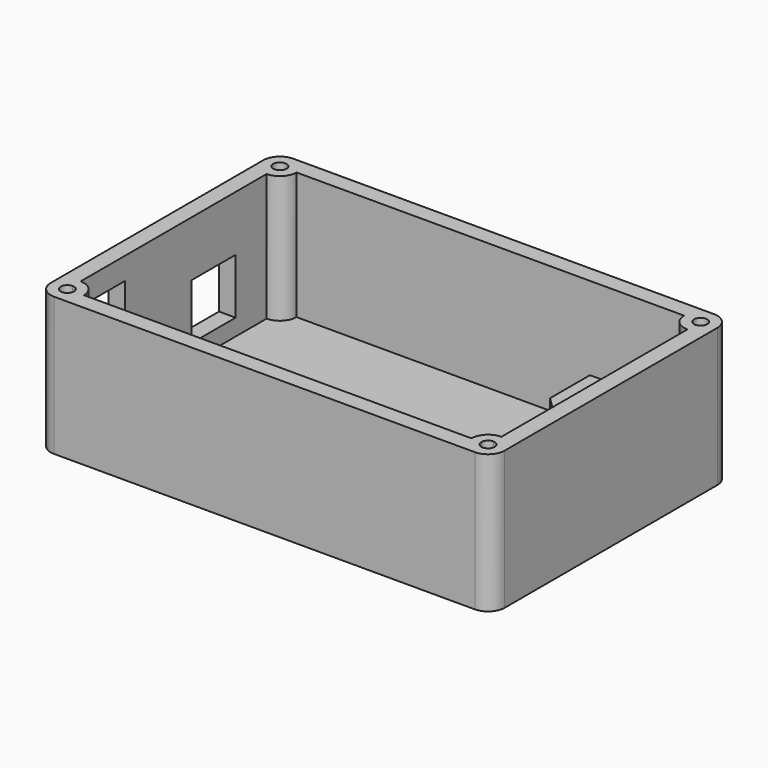
from build123d import *

# Parameters (mm, degrees)
F0_W     = 104.14
F0_H     = 68.58
F1_DEPTH = 31.75
F2_DEPTH = 12.7
F3_DEPTH = 2.54
F4_W     = 12.7
F4_H     = 12.7
F4_W_2   = 11.43
F4_H_2   = 20.32
F5_DEPTH = 10.16
F6_R     = 3.81
F7_R     = 3.80999
F8_DEPTH = 12.7


# Not quite as in the source:
# - a fillet or chamfer is up to 0.001 mm smaller than in the source, because OpenCascade refuses the exact size


with BuildPart() as f1:
    # F0 (on Top) → F1 (new body)
    with BuildSketch(Plane.XY):
        Rectangle(F0_W, F0_H)
        with BuildLine():
            ThreePointArc((-48.26, 28.956), (-49.3376307345, 31.5576307345), (-46.736, 30.48))
            Line((-46.736, 30.48), (-44.45, 30.48))
            Line((-44.45, 30.48), (22.86, 30.48))
            Line((22.86, 30.48), (25.4, 30.48))
            Line((25.4, 30.48), (44.45, 30.48))
            Line((44.45, 30.48), (46.736, 30.48))
            ThreePointArc((46.736, 30.48), (48.26, 32.004), (49.784, 30.48))
            ThreePointArc((49.784, 30.48), (49.3376307345, 29.4023692655), (48.26, 28.956))
            Line((48.26, 28.956), (48.26, 26.67))
            Line((48.26, 26.67), (48.26, -26.67))
            Line((48.26, -26.67), (48.26, -28.956))
            ThreePointArc((48.26, -28.956), (49.3376307345, -29.4023692655), (49.784, -30.48))
            ThreePointArc((49.784, -30.48), (48.26, -32.004), (46.736, -30.48))
            Line((46.736, -30.48), (44.45, -30.48))
            Line((44.45, -30.48), (25.4, -30.48))
            Line((25.4, -30.48), (22.86, -30.48))
            Line((22.86, -30.48), (-44.45, -30.48))
            Line((-44.45, -30.48), (-46.736, -30.48))
            ThreePointArc((-46.736, -30.48), (-49.3376307345, -31.5576307345), (-48.26, -28.956))
            Line((-48.26, -28.956), (-48.26, -26.67))
            Line((-48.26, -26.67), (-48.26, 26.67))
            Line((-48.26, 26.67), (-48.26, 28.956))
        make_face(mode=Mode.SUBTRACT)
        with BuildLine():
            Line((46.736, 30.48), (44.45, 30.48))
            Line((44.45, 30.48), (44.45, 26.67))
            Line((44.45, 26.67), (48.26, 26.67))
            Line((48.26, 26.67), (48.26, 28.956))
            ThreePointArc((48.26, 28.956), (47.1823692655, 29.4023692655), (46.736, 30.48))
        make_face()
        with BuildLine():
            Line((48.26, -28.956), (48.26, -26.67))
            Line((48.26, -26.67), (44.45, -26.67))
            Line((44.45, -26.67), (44.45, -30.48))
            Line((44.45, -30.48), (46.736, -30.48))
            ThreePointArc((46.736, -30.48), (47.1823692655, -29.4023692655), (48.26, -28.956))
        make_face()
        with BuildLine():
            Line((-44.45, -26.67), (-48.26, -26.67))
            Line((-48.26, -26.67), (-48.26, -28.956))
            ThreePointArc((-48.26, -28.956), (-47.1823692655, -29.4023692655), (-46.736, -30.48))
            Line((-46.736, -30.48), (-44.45, -30.48))
            Line((-44.45, -30.48), (-44.45, -26.67))
        make_face()
        with BuildLine():
            Line((-44.45, 30.48), (-46.736, 30.48))
            ThreePointArc((-46.736, 30.48), (-47.1823692655, 29.4023692655), (-48.26, 28.956))
            Line((-48.26, 28.956), (-48.26, 26.67))
            Line((-48.26, 26.67), (-44.45, 26.67))
            Line((-44.45, 26.67), (-44.45, 30.48))
        make_face()
    extrude(amount=F1_DEPTH)

    # F0 (on Top) → F2 (join)
    with BuildSketch(Plane.XY):
        Polygon((25.4, 30.48), (22.86, 30.48), (22.86, 19.05), (26.67, 15.24), (26.67, -24.13), (22.86, -27.94), (22.86, -30.48), (25.4, -30.48), (25.4, -27.94), (29.21, -24.13), (29.21, 15.24), (25.4, 19.05), align=None)
    extrude(amount=F2_DEPTH)

    # F0 (on Top) → F3 (join)
    with BuildSketch(Plane.XY):
        Polygon((22.86, 30.48), (-44.45, 30.48), (-44.45, 26.67), (-48.26, 26.67), (-48.26, -26.67), (-44.45, -26.67), (-44.45, -30.48), (22.86, -30.48), (22.86, -27.94), (26.67, -24.13), (26.67, 15.24), (22.86, 19.05), align=None)
        Polygon((44.45, 30.48), (25.4, 30.48), (25.4, 19.05), (29.21, 15.24), (29.21, -24.13), (25.4, -27.94), (25.4, -30.48), (44.45, -30.48), (44.45, -26.67), (48.26, -26.67), (48.26, 26.67), (44.45, 26.67), align=None)
    extrude(amount=F3_DEPTH)

    # F4 (on face) → F5 (cut)
    with BuildSketch(Plane(origin=(-52.07, 0, 0), x_dir=(0, -1, 0), z_dir=(-1, 0, 0))):
        with Locations((-11.43, 12.7)):
            Rectangle(F4_W, F4_H)
        with Locations((19.685, 16.51)):
            Rectangle(F4_W_2, F4_H_2)
    extrude(amount=-F5_DEPTH, mode=Mode.SUBTRACT)

    # F6
    f6_edges = [f1.edges().sort_by_distance(p)[0] for p in [
        (-52.07, -34.29, 15.875),
        (52.07, -34.29, 15.875),
        (52.07, 34.29, 15.875),
        (-52.07, 34.29, 15.875),
    ]]
    fillet(f6_edges, radius=F6_R)

    # F7 (radius 3.81 in the source; OpenCascade refuses exactly that, so slightly less here)
    f7_edges = [f1.edges().sort_by_distance(p)[0] for p in [
        (44.45, 26.67, 17.145),
        (-44.45, 26.67, 17.145),
        (44.45, -26.67, 17.145),
        (-44.45, -26.67, 17.145),
    ]]
    fillet(f7_edges, radius=F7_R)

    # F0 (on Top) → F8 (join)
    with BuildSketch(Plane.XY):
        with BuildLine():
            Line((-48.26, 28.956), (-48.26, 30.48))
            Line((-48.26, 30.48), (-46.736, 30.48))
            ThreePointArc((-46.736, 30.48), (-49.3376307345, 31.5576307345), (-48.26, 28.956))
        make_face()
        with BuildLine():
            Line((48.26, 30.48), (46.736, 30.48))
            ThreePointArc((46.736, 30.48), (47.1823692655, 29.4023692655), (48.26, 28.956))
            Line((48.26, 28.956), (48.26, 30.48))
        make_face()
        with BuildLine():
            ThreePointArc((49.784, 30.48), (48.26, 32.004), (46.736, 30.48))
            Line((46.736, 30.48), (48.26, 30.48))
            Line((48.26, 30.48), (48.26, 28.956))
            ThreePointArc((48.26, 28.956), (49.3376307345, 29.4023692655), (49.784, 30.48))
        make_face()
        with BuildLine():
            Line((-46.736, 30.48), (-48.26, 30.48))
            Line((-48.26, 30.48), (-48.26, 28.956))
            ThreePointArc((-48.26, 28.956), (-47.1823692655, 29.4023692655), (-46.736, 30.48))
        make_face()
        with BuildLine():
            Line((-48.26, -30.48), (-48.26, -28.956))
            ThreePointArc((-48.26, -28.956), (-49.3376307345, -31.5576307345), (-46.736, -30.48))
            Line((-46.736, -30.48), (-48.26, -30.48))
        make_face()
        with BuildLine():
            ThreePointArc((-46.736, -30.48), (-47.1823692655, -29.4023692655), (-48.26, -28.956))
            Line((-48.26, -28.956), (-48.26, -30.48))
            Line((-48.26, -30.48), (-46.736, -30.48))
        make_face()
        with BuildLine():
            ThreePointArc((49.784, -30.48), (49.3376307345, -29.4023692655), (48.26, -28.956))
            Line((48.26, -28.956), (48.26, -30.48))
            Line((48.26, -30.48), (46.736, -30.48))
            ThreePointArc((46.736, -30.48), (48.26, -32.004), (49.784, -30.48))
        make_face()
        with BuildLine():
            Line((48.26, -30.48), (48.26, -28.956))
            ThreePointArc((48.26, -28.956), (47.1823692655, -29.4023692655), (46.736, -30.48))
            Line((46.736, -30.48), (48.26, -30.48))
        make_face()
    extrude(amount=F8_DEPTH)


solid = f1.part
